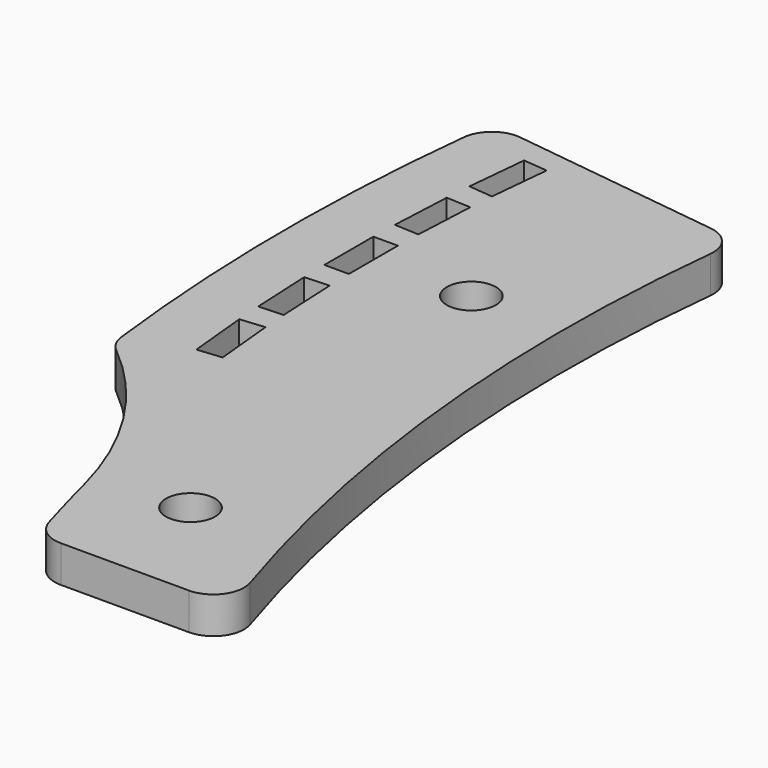
from build123d import *

# Parameters (mm, degrees)
F0_W        = 50.8
F0_H        = 127
F0_R        = 50.8
F1_DEPTH    = 76.2
F2_T1_DEPTH = 76.2
F3_R        = 63.5


# Not quite as in the source:
# - a fillet or chamfer that OpenCascade refuses, or shapes differently, is made with other operations: its cross-section is extruded or revolved along the edge and cut away or added
# - a feature names something its author has since deleted; it is built from what else it names


with BuildPart() as f1:
    # F0 (on Top) → F1 (new body)
    with BuildSketch(Plane.XY):
        with BuildLine():
            Line((-3842.1031233725, -492.1847614173), (-3653.1472320591, -467.9789534788))
            ThreePointArc((-3653.1472320591, -467.9789534788), (-3683, 0), (-3653.1472320591, 467.9789534788))
            Line((-3653.1472320591, 467.9789534788), (-3842.1031233725, 492.1847614173))
            ThreePointArc((-3842.1031233725, 492.1847614173), (-3873.5, 0), (-3842.1031233725, -492.1847614173))
        make_face()
        Polygon((-3672.3184884479, -419.8900563283), (-3722.8813354916, -424.7929635108), (-3735.1386034477, -298.3858459017), (-3684.5757564041, -293.4829387192), align=None, mode=Mode.SUBTRACT)
        Polygon((-3688.3163611044, -241.9776031163), (-3739.0570382274, -244.4319227962), (-3745.1928374272, -117.5802299885), (-3694.4521603041, -115.1259103086), align=None, mode=Mode.SUBTRACT)
        with Locations((-3721.1, 0)):
            Rectangle(F0_W, F0_H, mode=Mode.SUBTRACT)
        Polygon((-3694.4521603041, 115.1259103086), (-3745.1928374272, 117.5802299885), (-3739.0570382274, 244.4319227962), (-3688.3163611044, 241.9776031163), align=None, mode=Mode.SUBTRACT)
        Polygon((-3684.5757564041, 293.4829387192), (-3735.1386034477, 298.3858459017), (-3722.8813354916, 424.7929635108), (-3672.3184884479, 419.8900563283), align=None, mode=Mode.SUBTRACT)
        with BuildLine():
            Line((-3653.1472320591, -467.9789534788), (-3275.2354494323, -419.5673376017))
            ThreePointArc((-3275.2354494323, -419.5673376016), (-3302, 0), (-3275.2354494323, 419.5673376016))
            Line((-3275.2354494323, 419.5673376017), (-3653.1472320591, 467.9789534788))
            ThreePointArc((-3653.1472320591, 467.9789534788), (-3683, 0), (-3653.1472320591, -467.9789534788))
        make_face()
        with Locations((-3492.5, 0)):
            Circle(F0_R, mode=Mode.SUBTRACT)
        with BuildLine():
            Line((-3627.8456416998, -635), (-3240.367108832, -635))
            ThreePointArc((-3240.367108832, -635), (-3259.5815655268, -527.5718128161), (-3275.2354494323, -419.5673376016))
            Line((-3275.2354494323, -419.5673376017), (-3653.1472320591, -467.9789534788))
            ThreePointArc((-3653.1472320591, -467.9789534788), (-3641.4541483351, -551.6345579938), (-3627.8456416998, -635))
        make_face()
        with BuildLine():
            Line((-3517.3268486167, -1092.2), (-3116.1359341338, -1092.2))
            ThreePointArc((-3116.1359341338, -1092.2000000001), (-3186.4620967161, -865.8309917021), (-3240.367108832, -635))
            Line((-3240.367108832, -635), (-3627.8456416998, -635))
            ThreePointArc((-3627.8456416998, -635), (-3579.8925178131, -865.3661426853), (-3517.3268486167, -1092.1999999999))
        make_face()
        with Locations((-3384.0436300379, -863.6)):
            Circle(F0_R, mode=Mode.SUBTRACT)
    extrude(amount=F1_DEPTH)

    # F2: fillet of radius 762 on 1 edges, made by hand

    # F2_s2 → F2_t1 (join)
    with BuildSketch(Plane.XY):
        with BuildLine():
            ThreePointArc((-3842.1031233725, -492.1847614173), (-3670.9916584142, -676.9720156234), (-3569.4589749529, -907.4423541626))
            Line((-3569.4589749529, -907.4423541626), (-3554.6887998841, -903.6874202833))
            ThreePointArc((-3554.6887998841, -903.6874202833), (-3603.0108161093, -686.1315301017), (-3638.030760754, -466.0424888437))
            Line((-3638.030760754, -466.0424888437), (-3655.0836966942, -452.8624821737))
            ThreePointArc((-3655.0836966942, -452.8624821737), (-3749.5616423509, -464.965386143), (-3832.7858312721, -480.1246756831))
            Line((-3832.7858312721, -480.1246756831), (-3842.1031233725, -492.1847614173))
        make_face()
    extrude(amount=F2_T1_DEPTH)

    # F3
    f3_edges = [f1.edges().sort_by_distance(p)[0] for p in [
        (-3842.103123, -492.184761, 38.1),
        (-3842.103123, 492.184761, 38.1),
        (-3275.235449, 419.567338, 38.1),
        (-3116.135934, -1092.2, 38.1),
        (-3517.326849, -1092.2, 38.1),
    ]]
    fillet(f3_edges, radius=F3_R)


solid = f1.part
